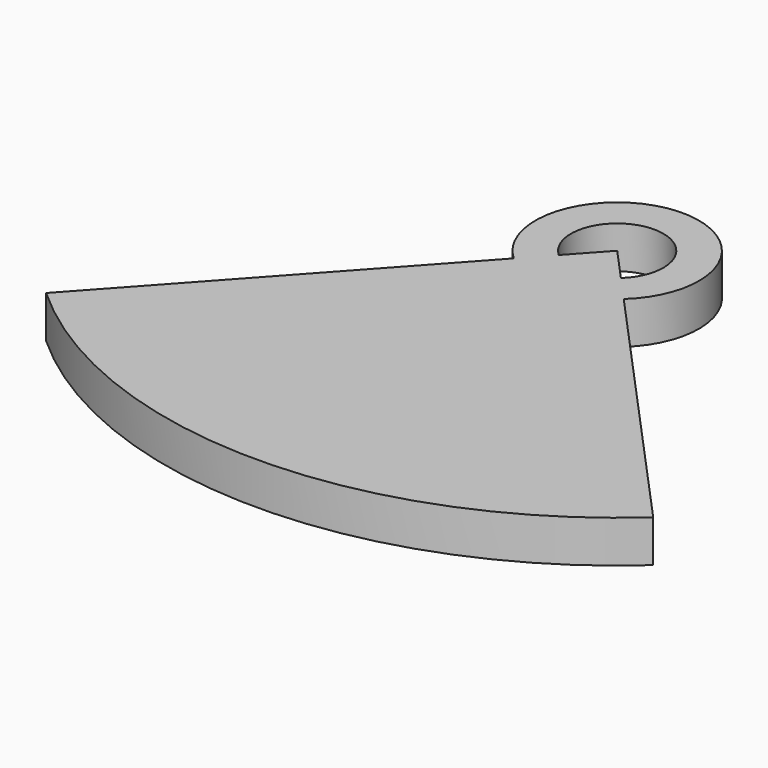
from build123d import *

# Parameters (mm, degrees)
F1_DEPTH = 3
F6_DEPTH = 3


# Not quite as in the source:
# - the program builds the solid bodies; features that only make, move or delete a surface that nothing else refers to are left out


with BuildPart() as f1:
    # F0 (on Top) → F1 (new body)
    with BuildSketch(Plane.XY):
        with BuildLine():
            Line((-3.8056071322, 19.4965880074), (-21.5033702552, 0))
            ThreePointArc((-21.5033702552, 0), (0.1091537997, -8.3463338313), (21.7216778547, 0))
            Line((21.7216778547, 0), (4.0239147316, 19.4965880074))
            Line((4.0239147316, 19.4965880074), (2.3194467965, 21.374300398))
            Line((2.3194467965, 21.374300398), (0.1091537997, 23.8092506024))
            Line((0.1091537997, 23.8092506024), (-2.1011391971, 21.374300398))
            Line((-2.1011391971, 21.374300398), (-3.8056071322, 19.4965880074))
        make_face()
        with BuildLine():
            Line((-15.8273540437, 0), (0.1091537997, 23.8092506024))
            Line((0.1091537997, 23.8092506024), (16.0456616431, 0))
            ThreePointArc((16.0456616431, 0), (0.1091537997, -4.8412763821), (-15.8273540437, 0))
        make_face(mode=Mode.SUBTRACT)
        with BuildLine():
            Line((16.0456616431, 0), (0.1091537997, 23.8092506024))
            Line((0.1091537997, 23.8092506024), (-15.8273540437, 0))
            ThreePointArc((-15.8273540437, 0), (0.1091537997, -4.8412763821), (16.0456616431, 0))
        make_face()
        with BuildLine():
            Line((-10.592116043, 0), (0.1091537997, 23.8092506024))
            Line((0.1091537997, 23.8092506024), (11.3627482206, 0))
            ThreePointArc((11.3627482206, 0), (0.3853160888, -2.256488537), (-10.592116043, 0))
        make_face(mode=Mode.SUBTRACT)
        with BuildLine():
            Line((11.3627482206, 0), (0.1091537997, 23.8092506024))
            Line((0.1091537997, 23.8092506024), (-10.592116043, 0))
            ThreePointArc((-10.592116043, 0), (0.3853160888, -2.256488537), (11.3627482206, 0))
        make_face()
    extrude(amount=F1_DEPTH)

    # F0 (on Top) → F6 (join)
    with BuildSketch(Plane.XY):
        with BuildLine():
            ThreePointArc((4.0239147316, 19.4965880074), (0.1091537997, 29.6337172572), (-3.8056071322, 19.4965880074))
            Line((-3.8056071322, 19.4965880074), (-2.1011391971, 21.374300398))
            ThreePointArc((-2.1011391971, 21.374300398), (0.1091537997, 27.0977727066), (2.3194467965, 21.374300398))
            Line((2.3194467965, 21.374300398), (4.0239147316, 19.4965880074))
        make_face()
    extrude(amount=F6_DEPTH)


solid = f1.part
